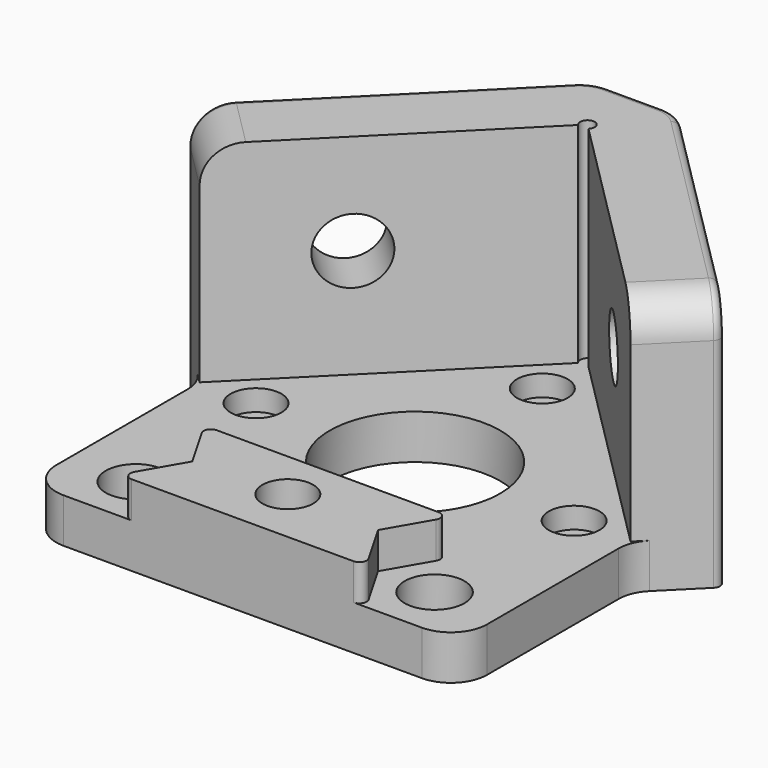
from build123d import *

# Parameters (mm, degrees)
F0_R          = 4.125
F0_R_2        = 1.7
F0_R_3        = 11.75
F1_DEPTH      = 6.13
F3_DEPTH      = 35
F4_R          = 4.5
F5_DEPTH      = 10
F6_R          = 4.25
F7_DEPTH      = 10
F8_R          = 7
F9_DEPTH      = 3
F10_R         = 7
F11_DEPTH     = 3
F13_R         = 5
F12_R         = 3.5
F14_DEPTH     = 2.9
F15_TEXT_SIZE = 7.1642815932
F16_DEPTH     = 0.25
F17_R         = 3.5
F18_DEPTH     = 5
F19_T1_DEPTH  = 32.5
F19_T3_DEPTH  = 9.3301270189
F19_T5_DEPTH  = 36.6690475583
F19_T7_DEPTH  = 7.5391052434
F19_T9_DEPTH  = 36.6690475583
F19_T12_ANGLE = 90
F19_T14_ANGLE = 45
F19_T16_ANGLE = 45
F19_T18_ANGLE = 90
F20_R         = 1
F21_DEPTH     = 28.87


# Not quite as in the source:
# - a fillet or chamfer that OpenCascade refuses, or shapes differently, is made with other operations: its cross-section is extruded or revolved along the edge and cut away or added
# - Text() gives the source's letters only with a copy of the font that has no kerning and outlines rounded to 1/6400 em; it was checked with that copy


with BuildPart() as f1:
    # F0 (on Top) → F1 (new body)
    with BuildSketch(Plane.XY):
        Polygon((-29.6984848098, 0), (0, 0), (29.6984848098, 0), (29.6984848098, 29.7), (0, 59.3984848098), (-29.6984848098, 29.7), align=None)
        with Locations((-20.59, 7.3196897832)):
            Circle(F0_R, mode=Mode.SUBTRACT)
        with Locations((0, 7.7796897832)):
            Circle(F0_R_2, mode=Mode.SUBTRACT)
        with Locations((20.59, 7.3196897832)):
            Circle(F0_R, mode=Mode.SUBTRACT)
        with Locations((-21.9203102168, 29.7)):
            Circle(F0_R_2, mode=Mode.SUBTRACT)
        with Locations((0, 29.7)):
            Circle(F0_R_3, mode=Mode.SUBTRACT)
        with Locations((21.9203102168, 29.7)):
            Circle(F0_R_2, mode=Mode.SUBTRACT)
        with Locations((0, 51.6203102168)):
            Circle(F0_R_2, mode=Mode.SUBTRACT)
    extrude(amount=F1_DEPTH)

    # F2 (on face) → F3 (join)
    with BuildSketch(Plane(origin=(0, 0, 0), x_dir=(1, 0, 0), z_dir=(0, 0, -1))):
        Polygon((0, -59.3984848098), (-29.6984848098, -29.7), (-36.7695526217, -36.7710678119), (-5.8406204336, -67.7), (0, -67.7), (5.8406204336, -67.7), (36.7695526217, -36.7710678119), (29.6984848098, -29.7), align=None)
    extrude(amount=-F3_DEPTH)

    # F4 (on face) → F5 (cut, through all)
    with BuildSketch(Plane(origin=(-29.6992424049, 29.6992424049, 0), x_dir=(0.7071067812, 0.7071067812, 0), z_dir=(0.7071067812, -0.7071067812, 0))):
        with Locations((16.6010714012, 21.13)):
            Circle(F4_R)
    extrude(amount=-F5_DEPTH, mode=Mode.SUBTRACT)

    # F6 (on face) → F7 (cut, through all)
    with BuildSketch(Plane(origin=(29.6992424049, 29.6992424049, 0), x_dir=(0.7071067812, -0.7071067812, 0), z_dir=(-0.7071067812, -0.7071067812, 0))):
        with Locations((-16.6010714012, 21.13)):
            Circle(F6_R)
    extrude(amount=-F7_DEPTH, mode=Mode.SUBTRACT)

    # F8 (on face) → F9 (cut)
    with BuildSketch(Plane(origin=(-36.7703102168, 36.7703102168, 0), x_dir=(-0.7071067812, -0.7071067812, 0), z_dir=(-0.7071067812, 0.7071067812, 0))):
        with Locations((-16.6010714006, 21.13)):
            Circle(F8_R)
    extrude(amount=-F9_DEPTH, mode=Mode.SUBTRACT)

    # F10 (on face) → F11 (cut)
    with BuildSketch(Plane(origin=(36.7703102168, 36.7703102168, 0), x_dir=(-0.7071067812, 0.7071067812, 0), z_dir=(0.7071067812, 0.7071067812, 0))):
        with Locations((16.6010714007, 21.13)):
            Circle(F10_R)
    extrude(amount=-F11_DEPTH, mode=Mode.SUBTRACT)

    # F13
    f13_edges = [f1.edges().sort_by_distance(p)[0] for p in [
        (33.234019, 33.235534, 35),
        (-33.234019, 33.235534, 35),
        (29.698485, 29.7, 3.065),
        (29.698485, 0, 3.065),
        (-29.698485, 0, 3.065),
        (-29.698485, 29.7, 3.065),
        (-5.84062, 67.7, 17.5),
        (5.84062, 67.7, 17.5),
    ]]
    fillet(f13_edges, radius=F13_R)

    # F12 (on face) → F14 (cut)
    with BuildSketch(Plane.XY.offset(6.13)):
        with Locations((0, 51.6203102168)):
            Circle(F12_R)
        with Locations((-21.9203102168, 29.7)):
            Circle(F12_R)
        with Locations((21.9203102168, 29.7)):
            Circle(F12_R)
        with Locations((0, 7.7796897832)):
            Circle(F12_R)
    extrude(amount=-F14_DEPTH, mode=Mode.SUBTRACT)

    # F15 (on face) → F16 (cut)
    with BuildSketch(Plane(origin=(-36.7703102168, 36.7703102168, 0), x_dir=(-0.7071067812, -0.7071067812, 0), z_dir=(-0.7071067812, 0.7071067812, 0))):
        with Locations((-41.6701189596, 3.2)):
            Text('SIENCI LABS', F15_TEXT_SIZE, font='Open Sans', text_align=(TextAlign.LEFT, TextAlign.BOTTOM))
    extrude(amount=-F16_DEPTH, mode=Mode.SUBTRACT)

    # F17 (on face) → F18 (join)
    with BuildSketch(Plane.XY.offset(6.13)):
        Polygon((16.692885683, 14.0696897832), (-16.692885683, 14.0696897832), (-12.7957713659, 7.3196897832), (-16.692885683, 0.5696897832), (16.692885683, 0.5696897832), (12.7957713659, 7.3196897832), align=None)
        with Locations((0, 7.7796897832)):
            Circle(F17_R, mode=Mode.SUBTRACT)
        Polygon((16.692885683, 0.5696897832), (-16.692885683, 0.5696897832), (-17.0217962327, 0), (0, 0), (17.0217962327, 0), align=None)
        Polygon((-17.0217962327, 14.6393795664), (-16.692885683, 14.0696897832), (16.692885683, 14.0696897832), (17.0217962327, 14.6393795664), (0, 14.6393795664), align=None)
    extrude(amount=F18_DEPTH)

    # F19: fillet of radius 1 on 13 edges, made by hand

    # F19_s2 → F19_t1 (cut)
    with BuildSketch(Plane.XY.offset(-2.5)):
        with BuildLine():
            ThreePointArc((36.0624458405, 37.4781745931), (36.3553390593, 36.7710678119), (36.0624458405, 36.0639610307))
            Line((36.0624458405, 36.0639610307), (36.7695526217, 36.7710678119))
            Line((36.7695526217, 36.7710678119), (36.0624458405, 37.4781745931))
        make_face()
        with BuildLine():
            ThreePointArc((-36.0624458405, 36.0639610307), (-36.3553390593, 36.7710678119), (-36.0624458405, 37.4781745931))
            Line((-36.0624458405, 37.4781745931), (-36.7695526217, 36.7710678119))
            Line((-36.7695526217, 36.7710678119), (-36.0624458405, 36.0639610307))
        make_face()
    extrude(amount=F19_T1_DEPTH, mode=Mode.SUBTRACT)

    # F19_s4 → F19_t3 (cut)
    with BuildSketch(Plane.XY.offset(6.13)):
        with BuildLine():
            ThreePointArc((-15.2897454251, 0), (-16.1557708289, 0.5), (-16.1557708289, 1.5))
            Line((-16.1557708289, 1.5), (-17.0217962327, 0))
            Line((-17.0217962327, 0), (-15.2897454251, 0))
        make_face()
        with BuildLine():
            ThreePointArc((-15.2897454251, 14.6393795664), (-16.1557708289, 14.1393795664), (-16.1557708289, 13.1393795664))
            Line((-16.1557708289, 13.1393795664), (-17.0217962327, 14.6393795664))
            Line((-17.0217962327, 14.6393795664), (-15.2897454251, 14.6393795664))
        make_face()
        with BuildLine():
            ThreePointArc((16.1557708289, 13.1393795664), (16.1557708289, 14.1393795664), (15.2897454251, 14.6393795664))
            Line((15.2897454251, 14.6393795664), (17.0217962327, 14.6393795664))
            Line((17.0217962327, 14.6393795664), (16.1557708289, 13.1393795664))
        make_face()
        with BuildLine():
            ThreePointArc((15.2897454251, 0), (16.1557708289, 0.5), (16.1557708289, 1.5))
            Line((16.1557708289, 1.5), (17.0217962327, 0))
            Line((17.0217962327, 0), (15.2897454251, 0))
        make_face()
    extrude(amount=F19_T3_DEPTH, mode=Mode.SUBTRACT)

    # F19_s6 → F19_t5 (cut)
    with BuildSketch(Plane(origin=(3.536291501, 3.536291501, 0), x_dir=(0, 0, 1), z_dir=(0.7071067812, 0.7071067812, 0))):
        with BuildLine():
            ThreePointArc((34, -52.0010714012), (34.7071067812, -51.7081781824), (35, -51.0010714012))
            Line((35, -51.0010714012), (35, -52.0010714012))
            Line((35, -52.0010714012), (34, -52.0010714012))
        make_face()
    extrude(amount=F19_T5_DEPTH, mode=Mode.SUBTRACT)

    # F19_s8 → F19_t7 (cut)
    with BuildSketch(Plane.YZ.offset(-3.7695526217)):
        with BuildLine():
            ThreePointArc((67.7, 34), (67.4071067812, 34.7071067812), (66.7, 35))
            Line((66.7, 35), (67.7, 35))
            Line((67.7, 35), (67.7, 34))
        make_face()
    extrude(amount=F19_T7_DEPTH, mode=Mode.SUBTRACT)

    # F19_s10 → F19_t9 (cut)
    with BuildSketch(Plane(origin=(-29.4652236891, 29.4652236891, 0), x_dir=(0, 0, 1), z_dir=(0.7071067812, -0.7071067812, 0))):
        with BuildLine():
            ThreePointArc((34, -52.0010714012), (34.7071067812, -51.7081781824), (35, -51.0010714012))
            Line((35, -51.0010714012), (35, -52.0010714012))
            Line((35, -52.0010714012), (34, -52.0010714012))
        make_face()
    extrude(amount=F19_T9_DEPTH, mode=Mode.SUBTRACT)

    # F19_s11 → F19_t12 (revolve, cut)
    with BuildSketch(Plane.XY.offset(30)):
        with BuildLine():
            ThreePointArc((-36.0624458405, 37.4781745931), (-36.3553390593, 36.7710678119), (-36.0624458405, 36.0639610307))
            Line((-36.0624458405, 36.0639610307), (-36.7695526217, 36.7710678119))
            Line((-36.7695526217, 36.7710678119), (-36.0624458405, 37.4781745931))
        make_face()
    revolve(axis=Axis((-33.2340187158, 40.3066017178, 30), (-0.7071067812, 0.7071067812, 0)), revolution_arc=F19_T12_ANGLE, mode=Mode.SUBTRACT)

    # F19_s13 → F19_t14 (revolve, cut)
    with BuildSketch(Plane.YZ.offset(-3.7695526217)):
        with BuildLine():
            ThreePointArc((67.7, 34), (67.4071067812, 34.7071067812), (66.7, 35))
            Line((66.7, 35), (67.7, 35))
            Line((67.7, 35), (67.7, 34))
        make_face()
    revolve(axis=Axis((-3.7695526217, 62.7, 35), (0, 0, 1)), revolution_arc=F19_T14_ANGLE, mode=Mode.SUBTRACT)

    # F19_s15 → F19_t16 (revolve, cut)
    with BuildSketch(Plane(origin=(-29.4652236891, 29.4652236891, 0), x_dir=(0, 0, 1), z_dir=(0.7071067812, -0.7071067812, 0))):
        with BuildLine():
            ThreePointArc((34, -52.0010714012), (34.7071067812, -51.7081781824), (35, -51.0010714012))
            Line((35, -51.0010714012), (35, -52.0010714012))
            Line((35, -52.0010714012), (34, -52.0010714012))
        make_face()
    revolve(axis=Axis((3.7695526217, 62.7, 35), (0, 0, 1)), revolution_arc=F19_T16_ANGLE, mode=Mode.SUBTRACT)

    # F19_s17 → F19_t18 (revolve, cut)
    with BuildSketch(Plane.XY.offset(30)):
        with BuildLine():
            ThreePointArc((36.0624458405, 37.4781745931), (36.3553390593, 36.7710678119), (36.0624458405, 36.0639610307))
            Line((36.0624458405, 36.0639610307), (36.7695526217, 36.7710678119))
            Line((36.7695526217, 36.7710678119), (36.0624458405, 37.4781745931))
        make_face()
    revolve(axis=Axis((33.2340187158, 40.3066017178, 30), (-0.7071067812, -0.7071067812, 0)), revolution_arc=F19_T18_ANGLE, mode=Mode.SUBTRACT)

    # F20 (on face) → F21 (cut, through all)
    with BuildSketch(Plane.XY.offset(35)):
        with Locations((0, 59.3984848098)):
            Circle(F20_R)
    extrude(amount=-F21_DEPTH, mode=Mode.SUBTRACT)


solid = f1.part
